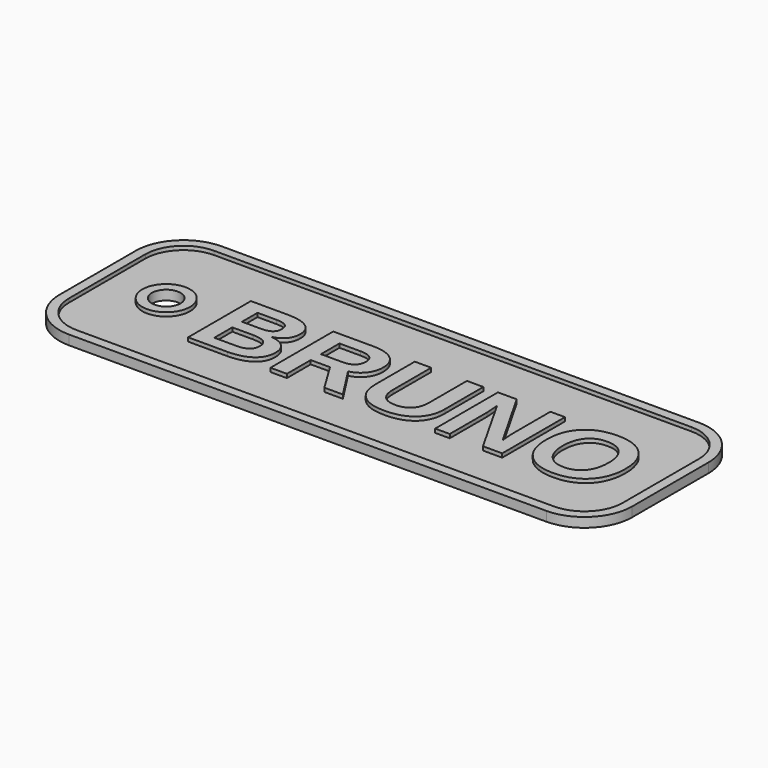
from build123d import *

# Parameters (mm, degrees)
F0_W         = 60
F0_H         = 20
F1_DEPTH     = 1
F2_R         = 5
F3_R         = 2.5
F4_DEPTH     = 0.4
F5_R         = 1.5
F6_DEPTH     = 1.001
F7_TEXT_SIZE = 11.9444444444
F8_DEPTH     = 0.4


# Not quite as in the source:
# - Text() gives the source's letters only with a copy of the font that has no kerning and outlines rounded to 1/6400 em; it was checked with that copy


with BuildPart() as f1:
    # F0 (on Top) → F1 (new body)
    with BuildSketch(Plane.XY):
        Rectangle(F0_W, F0_H)
    extrude(amount=F1_DEPTH)

    # F2
    f2_edges = [f1.edges().sort_by_distance(p)[0] for p in [
        (-30, -10, 0.5),
        (30, -10, 0.5),
        (30, 10, 0.5),
        (-30, 10, 0.5),
    ]]
    fillet(f2_edges, radius=F2_R)

    # F3 (on face) → F4 (cut)
    with BuildSketch(Plane.XY.offset(1)):
        with BuildLine():
            ThreePointArc((29, 5), (27.8284271247, 7.8284271247), (25, 9))
            Line((25, 9), (-25, 9))
            ThreePointArc((-25, 9), (-27.8284271247, 7.8284271247), (-29, 5))
            Line((-29, 5), (-29, -5))
            ThreePointArc((-29, -5), (-27.8284271247, -7.8284271247), (-25, -9))
            Line((-25, -9), (25, -9))
            ThreePointArc((25, -9), (27.8284271247, -7.8284271247), (29, -5))
            Line((29, -5), (29, 5))
        make_face()
        with Locations((-22.8122994304, 0)):
            Circle(F3_R, mode=Mode.SUBTRACT)
    extrude(amount=-F4_DEPTH, mode=Mode.SUBTRACT)

    # F5 (on face) → F6 (cut, through all)
    with BuildSketch(Plane.XY.offset(1)):
        with Locations((-22.8122994304, 0)):
            Circle(F5_R)
    extrude(amount=-F6_DEPTH, mode=Mode.SUBTRACT)

    # F7 (on face) → F8 (join)
    with BuildSketch(Plane.XY.offset(0.6)):
        with Locations((-17.8770507888, -4.3)):
            Text('BRUNO', F7_TEXT_SIZE, font='Arimo', font_style=FontStyle.BOLD, text_align=(TextAlign.LEFT, TextAlign.BOTTOM))
    extrude(amount=F8_DEPTH)


solid = f1.part
